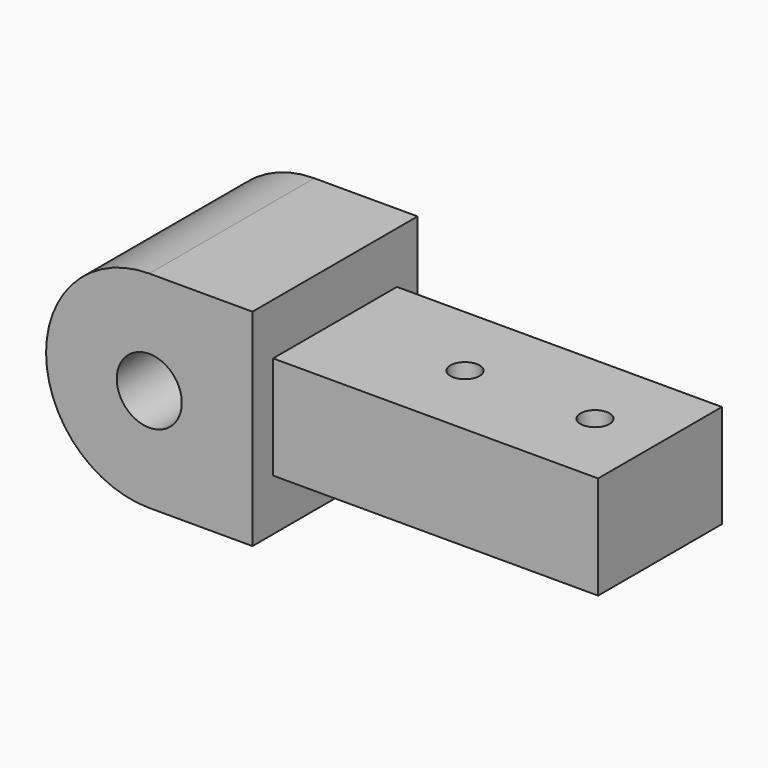
from build123d import *

# Parameters (mm, degrees)
F0_W     = 40
F0_H     = 19.05
F1_DEPTH = 12.7
F2_W     = 25.4
F2_H     = 25.4
F2_W_2   = 19.05
F2_H_2   = 12.7
F3_DEPTH = 25.4
F5_D     = 8
F6_R     = 12.69999
F8_D     = 3.571875


# Not quite as in the source:
# - a fillet or chamfer is up to 0.001 mm smaller than in the source, because OpenCascade refuses the exact size


with BuildPart() as f1:
    # F0 (on Top) → F1 (new body)
    with BuildSketch(Plane.XY):
        Rectangle(F0_W, F0_H)
    extrude(amount=F1_DEPTH)

    # F2 (on face) → F3 (join)
    with BuildSketch(Plane(origin=(-20, 0, 0), x_dir=(0, -1, 0), z_dir=(-1, 0, 0))):
        with Locations((0, 6.35)):
            Rectangle(F2_W, F2_H)
        with Locations((0, 6.35)):
            Rectangle(F2_W_2, F2_H_2, mode=Mode.SUBTRACT)
        with Locations((0, 6.35)):
            Rectangle(F2_W_2, F2_H_2)
    extrude(amount=F3_DEPTH)

    # F5 (through all)
    with Locations(Plane.XZ.offset(12.7)):
        with Locations((-32.7, 6.35)):
            Hole(F5_D / 2)

    # F6 (radius 12.7 in the source; OpenCascade refuses exactly that, so slightly less here)
    f6_edges = [f1.edges().sort_by_distance(p)[0] for p in [
        (-45.4, 0, 19.05),
        (-45.4, 0, -6.35),
    ]]
    fillet(f6_edges, radius=F6_R)

    # F8 (through all)
    with Locations(Plane.XY.offset(12.7)):
        with Locations((12, 0), (-4, 0)):
            Hole(F8_D / 2)


solid = f1.part
